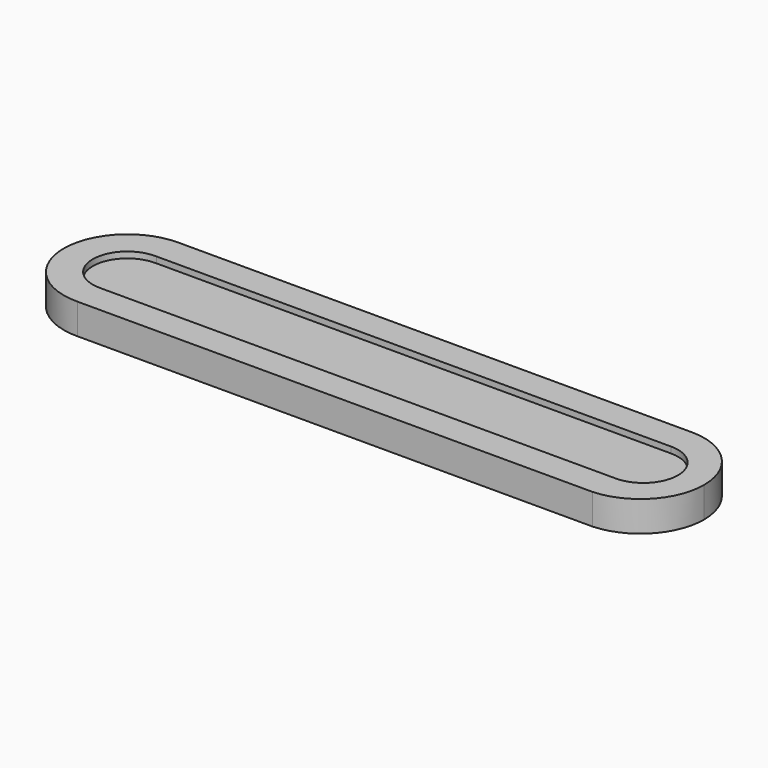
from build123d import *

# Parameters (mm, degrees)
F1_DEPTH = 3.81
F2_DEPTH = 3.048


with BuildPart() as f1:
    # F0 (on Top) → F1 (new body)
    with BuildSketch(Plane.XY):
        with BuildLine():
            ThreePointArc((-19.510121746, 6.3950662109), (-22.3157867582, 9.0185520845), (-26.0244197252, 10.0187899587))
            Line((-26.0244197252, 10.0187899587), (-26.0244197252, 6.3950662109))
            Line((-26.0244197252, 6.3950662109), (-19.510121746, 6.3950662109))
        make_face()
        with BuildLine():
            Line((-26.0244197252, 6.3950662109), (-26.0244197252, 10.0187899587))
            ThreePointArc((-26.0244197252, 10.0187899587), (-34.1203354035, 2.0770662109), (-26.0244197252, -5.8646575368))
            Line((-26.0244197252, -5.8646575368), (-26.0244197252, -2.2382320992))
            ThreePointArc((-26.0244197252, -2.2382320992), (-30.4951433134, 2.0770662109), (-26.0244197252, 6.3923645211))
            Line((-26.0244197252, 6.3923645211), (-26.0244197252, 6.3950662109))
        make_face()
        with BuildLine():
            Line((37.4916443036, 10.0187899587), (-26.0244197252, 10.0187899587))
            ThreePointArc((-26.0244197252, 10.0187899587), (-22.3157867582, 9.0185520845), (-19.510121746, 6.3950662109))
            Line((-19.510121746, 6.3950662109), (31.1912137245, 6.3950662109))
            ThreePointArc((31.1912137245, 6.3950662109), (33.9031065879, 8.9690226069), (37.4916443036, 10.0187899587))
        make_face()
        with BuildLine():
            Line((38.2424543545, 10.0187899587), (37.4916443036, 10.0187899587))
            ThreePointArc((37.4916443036, 10.0187899587), (33.9031065879, 8.9690226069), (31.1912137245, 6.3950662109))
            Line((31.1912137245, 6.3950662109), (38.2424543545, 6.3950662109))
            Line((38.2424543545, 6.3950662109), (38.2424543545, 10.0187899587))
        make_face()
        with BuildLine():
            ThreePointArc((-19.5083727315, -2.2382320992), (-22.3143805661, -4.8636372504), (-26.0244197252, -5.8646575368))
            Line((-26.0244197252, -5.8646575368), (37.4916443036, -5.8646575368))
            ThreePointArc((37.4916443036, -5.8646575368), (33.9017122748, -4.8140880512), (31.1894670186, -2.2382320992))
            Line((31.1894670186, -2.2382320992), (-19.5083727315, -2.2382320992))
        make_face()
        with BuildLine():
            Line((-26.0244197252, -2.2382320992), (-26.0244197252, -5.8646575368))
            ThreePointArc((-26.0244197252, -5.8646575368), (-22.3143805661, -4.8636372504), (-19.5083727315, -2.2382320992))
            Line((-19.5083727315, -2.2382320992), (-26.0244197252, -2.2382320992))
        make_face()
        with BuildLine():
            ThreePointArc((45.8176408176, 2.0770662109), (43.6201614007, 7.5646527942), (38.2424543545, 10.0187899587))
            Line((38.2424543545, 10.0187899587), (38.2424543545, 6.3950662109))
            ThreePointArc((38.2424543545, 6.3950662109), (41.2957414356, 5.1303532921), (42.5604543545, 2.0770662109))
            ThreePointArc((42.5604543545, 2.0770662109), (41.2957414356, -0.9762208702), (38.2424543545, -2.2409337891))
            Line((38.2424543545, -2.2409337891), (38.2424543545, -5.8646575368))
            ThreePointArc((38.2424543545, -5.8646575368), (43.6201614007, -3.4105203724), (45.8176408176, 2.0770662109))
        make_face()
        with BuildLine():
            ThreePointArc((31.1894670186, -2.2382320992), (33.9017122748, -4.8140880512), (37.4916443036, -5.8646575368))
            Line((37.4916443036, -5.8646575368), (38.2424543545, -5.8646575368))
            Line((38.2424543545, -5.8646575368), (38.2424543545, -2.2409337891))
            ThreePointArc((38.2424543545, -2.2409337891), (38.1660806131, -2.2402583138), (38.0897307663, -2.2382320992))
            Line((38.0897307663, -2.2382320992), (31.1894670186, -2.2382320992))
        make_face()
    extrude(amount=F1_DEPTH)

    # F0 (on Top) → F2 (join)
    with BuildSketch(Plane.XY):
        with BuildLine():
            Line((37.4916443036, 10.0187899587), (-26.0244197252, 10.0187899587))
            ThreePointArc((-26.0244197252, 10.0187899587), (-22.3157867582, 9.0185520845), (-19.510121746, 6.3950662109))
            Line((-19.510121746, 6.3950662109), (31.1912137245, 6.3950662109))
            ThreePointArc((31.1912137245, 6.3950662109), (33.9031065879, 8.9690226069), (37.4916443036, 10.0187899587))
        make_face()
        with BuildLine():
            Line((31.1912137245, 6.3950662109), (-19.510121746, 6.3950662109))
            ThreePointArc((-19.510121746, 6.3950662109), (-18.5596721596, 4.3283844472), (-18.2339512233, 2.0770662109))
            ThreePointArc((-18.2339512233, 2.0770662109), (-18.5592162228, -0.1727087604), (-19.5083727315, -2.2382320992))
            Line((-19.5083727315, -2.2382320992), (31.1894670186, -2.2382320992))
            ThreePointArc((31.1894670186, -2.2382320992), (29.9164580032, 2.0786747903), (31.1912137245, 6.3950662109))
        make_face()
        with BuildLine():
            Line((38.2424543545, 10.0187899587), (37.4916443036, 10.0187899587))
            ThreePointArc((37.4916443036, 10.0187899587), (33.9031065879, 8.9690226069), (31.1912137245, 6.3950662109))
            Line((31.1912137245, 6.3950662109), (38.2424543545, 6.3950662109))
            Line((38.2424543545, 6.3950662109), (38.2424543545, 10.0187899587))
        make_face()
        with BuildLine():
            Line((38.2424543545, 6.3950662109), (31.1912137245, 6.3950662109))
            ThreePointArc((31.1912137245, 6.3950662109), (29.9164580032, 2.0786747903), (31.1894670186, -2.2382320992))
            Line((31.1894670186, -2.2382320992), (38.0897307663, -2.2382320992))
            ThreePointArc((38.0897307663, -2.2382320992), (33.9251298298, 2.1534399524), (38.2424543545, 6.3950662109))
        make_face()
        with BuildLine():
            Line((38.2424543545, -2.2382320992), (38.2424543545, 6.3950662109))
            ThreePointArc((38.2424543545, 6.3950662109), (33.9251298298, 2.1534399524), (38.0897307663, -2.2382320992))
            Line((38.0897307663, -2.2382320992), (38.2424543545, -2.2382320992))
        make_face()
        with BuildLine():
            ThreePointArc((42.5604543545, 2.0770662109), (41.2957414356, 5.1303532921), (38.2424543545, 6.3950662109))
            Line((38.2424543545, 6.3950662109), (38.2424543545, -2.2382320992))
            Line((38.2424543545, -2.2382320992), (38.2424543545, -2.2409337891))
            ThreePointArc((38.2424543545, -2.2409337891), (41.2957414356, -0.9762208702), (42.5604543545, 2.0770662109))
        make_face()
        with BuildLine():
            ThreePointArc((45.8176408176, 2.0770662109), (43.6201614007, 7.5646527942), (38.2424543545, 10.0187899587))
            Line((38.2424543545, 10.0187899587), (38.2424543545, 6.3950662109))
            ThreePointArc((38.2424543545, 6.3950662109), (41.2957414356, 5.1303532921), (42.5604543545, 2.0770662109))
            ThreePointArc((42.5604543545, 2.0770662109), (41.2957414356, -0.9762208702), (38.2424543545, -2.2409337891))
            Line((38.2424543545, -2.2409337891), (38.2424543545, -5.8646575368))
            ThreePointArc((38.2424543545, -5.8646575368), (43.6201614007, -3.4105203724), (45.8176408176, 2.0770662109))
        make_face()
        with BuildLine():
            ThreePointArc((31.1894670186, -2.2382320992), (33.9017122748, -4.8140880512), (37.4916443036, -5.8646575368))
            Line((37.4916443036, -5.8646575368), (38.2424543545, -5.8646575368))
            Line((38.2424543545, -5.8646575368), (38.2424543545, -2.2409337891))
            ThreePointArc((38.2424543545, -2.2409337891), (38.1660806131, -2.2402583138), (38.0897307663, -2.2382320992))
            Line((38.0897307663, -2.2382320992), (31.1894670186, -2.2382320992))
        make_face()
        with BuildLine():
            ThreePointArc((-19.5083727315, -2.2382320992), (-22.3143805661, -4.8636372504), (-26.0244197252, -5.8646575368))
            Line((-26.0244197252, -5.8646575368), (37.4916443036, -5.8646575368))
            ThreePointArc((37.4916443036, -5.8646575368), (33.9017122748, -4.8140880512), (31.1894670186, -2.2382320992))
            Line((31.1894670186, -2.2382320992), (-19.5083727315, -2.2382320992))
        make_face()
        with BuildLine():
            Line((-19.510121746, 6.3950662109), (-26.0244197252, 6.3950662109))
            Line((-26.0244197252, 6.3950662109), (-26.0244197252, 6.3923645211))
            ThreePointArc((-26.0244197252, 6.3923645211), (-23.0703294749, 5.0758712685), (-21.8591433134, 2.0770662109))
            ThreePointArc((-21.8591433134, 2.0770662109), (-23.0703294749, -0.9217388466), (-26.0244197252, -2.2382320992))
            Line((-26.0244197252, -2.2382320992), (-19.5083727315, -2.2382320992))
            ThreePointArc((-19.5083727315, -2.2382320992), (-18.5592162228, -0.1727087604), (-18.2339512233, 2.0770662109))
            ThreePointArc((-18.2339512233, 2.0770662109), (-18.5596721596, 4.3283844472), (-19.510121746, 6.3950662109))
        make_face()
        with BuildLine():
            Line((-26.0244197252, -2.2382320992), (-26.0244197252, 6.3923645211))
            ThreePointArc((-26.0244197252, 6.3923645211), (-30.4951433134, 2.0770662109), (-26.0244197252, -2.2382320992))
        make_face()
        with BuildLine():
            ThreePointArc((-21.8591433134, 2.0770662109), (-23.0703294749, 5.0758712685), (-26.0244197252, 6.3923645211))
            Line((-26.0244197252, 6.3923645211), (-26.0244197252, -2.2382320992))
            ThreePointArc((-26.0244197252, -2.2382320992), (-23.0703294749, -0.9217388466), (-21.8591433134, 2.0770662109))
        make_face()
        with BuildLine():
            ThreePointArc((-19.510121746, 6.3950662109), (-22.3157867582, 9.0185520845), (-26.0244197252, 10.0187899587))
            Line((-26.0244197252, 10.0187899587), (-26.0244197252, 6.3950662109))
            Line((-26.0244197252, 6.3950662109), (-19.510121746, 6.3950662109))
        make_face()
        with BuildLine():
            Line((-26.0244197252, -2.2382320992), (-26.0244197252, -5.8646575368))
            ThreePointArc((-26.0244197252, -5.8646575368), (-22.3143805661, -4.8636372504), (-19.5083727315, -2.2382320992))
            Line((-19.5083727315, -2.2382320992), (-26.0244197252, -2.2382320992))
        make_face()
    extrude(amount=F2_DEPTH)


solid = f1.part
